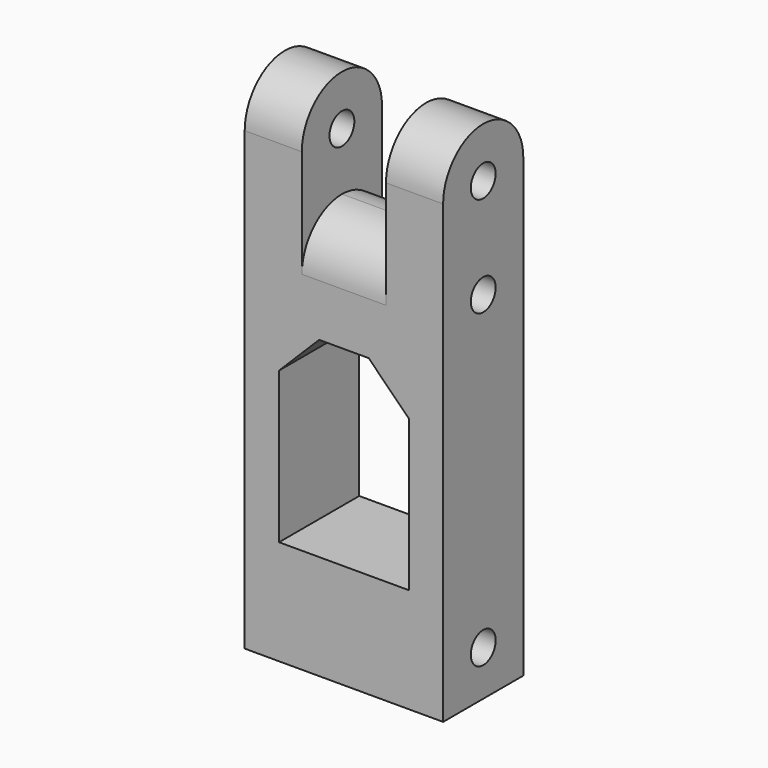
from build123d import *

# Parameters (mm, degrees)
F0_R     = 1.55
F1_DEPTH = 9.9
F2_W     = 8.4
F2_H     = 11.5120084733
F2_W_2   = 12.9466587678
F2_H_2   = 19.0824847668
F3_DEPTH = 25
F4_R     = 4.99999
F5_SIZE  = 4


# Not quite as in the source:
# - a fillet or chamfer is up to 0.001 mm smaller than in the source, because OpenCascade refuses the exact size
# - a feature names something its author has since deleted; it is built from what else it names


with BuildPart() as f1:
    # F0 (on Right) → F1 (new body, symmetric)
    with BuildSketch(Plane.YZ):
        with BuildLine():
            Line((-5, 25.5), (-5, -20))
            Line((-5, -20), (5, -20))
            Line((5, -20), (5, 25.5))
            Line((5, 25.5), (1.55, 25.5))
            ThreePointArc((1.55, 25.5), (0, 23.95), (-1.55, 25.5))
            Line((-1.55, 25.5), (-5, 25.5))
        make_face()
        with Locations((0, -15.5)):
            Circle(F0_R, mode=Mode.SUBTRACT)
        with Locations((0, 15.5)):
            Circle(F0_R, mode=Mode.SUBTRACT)
        with BuildLine():
            ThreePointArc((5, 25.5), (0, 30.5), (-5, 25.5))
            Line((-5, 25.5), (-1.55, 25.5))
            ThreePointArc((-1.55, 25.5), (0, 27.05), (1.55, 25.5))
            Line((1.55, 25.5), (5, 25.5))
        make_face()
    extrude(amount=F1_DEPTH, both=True)

    # F2 (on face) → F3 (cut)
    with BuildSketch(Plane.XZ.offset(5)):
        with Locations((0, 25.5)):
            Rectangle(F2_W, F2_H)
        Rectangle(F2_W_2, F2_H_2)
    extrude(amount=-F3_DEPTH, mode=Mode.SUBTRACT)

    # F4 (radius 5 in the source; OpenCascade refuses exactly that, so slightly less here)
    f4_edges = [f1.edges().sort_by_distance(p)[0] for p in [
        (0, -5, 19.743996),
        (0, 5, 19.743996),
    ]]
    fillet(f4_edges, radius=F4_R)

    # F5
    f5_edges = [f1.edges().sort_by_distance(p)[0] for p in [
        (6.473329, 0, 9.541242),
        (-6.473329, 0, 9.541242),
    ]]
    chamfer(f5_edges, length=F5_SIZE)


solid = f1.part
